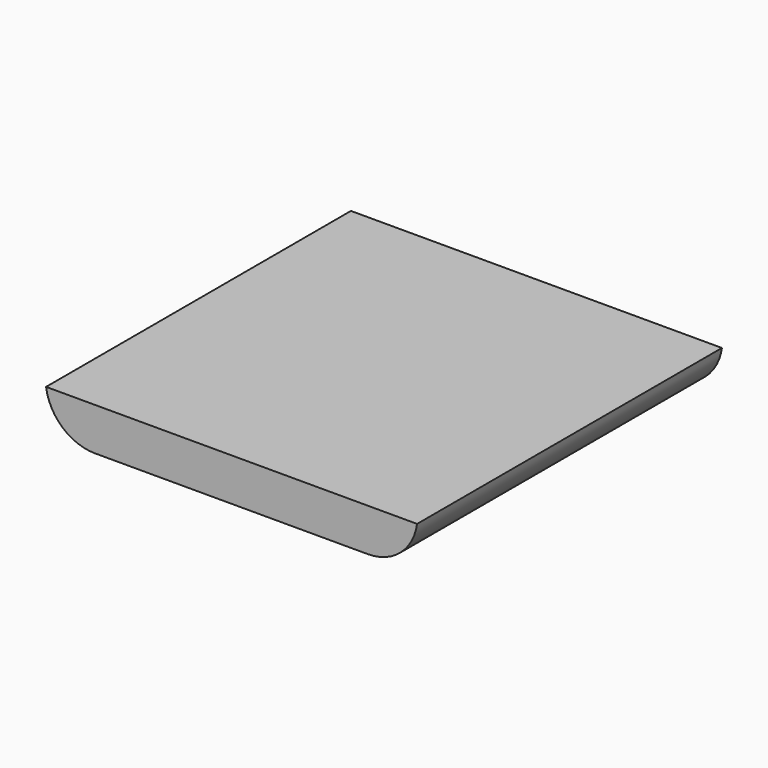
from build123d import *

# Parameters (mm, degrees)
F0_W        = 495.8
F0_H        = 509.2
F1_DEPTH    = 57
F2_T1_DEPTH = 836.1174207656


# Not quite as in the source:
# - a fillet or chamfer that OpenCascade refuses, or shapes differently, is made with other operations: its cross-section is extruded or revolved along the edge and cut away or added


with BuildPart() as f1:
    # F0 (on Top) → F1 (new body)
    with BuildSketch(Plane.XY):
        with Locations((247.9, -254.6)):
            Rectangle(F0_W, F0_H)
    extrude(amount=F1_DEPTH)

    # F2: fillet of radius 66 on 2 edges, made by hand

    # F2_s2 → F2_t1 (cut)
    with BuildSketch(Plane.XZ.offset(-163.4587103828)):
        with BuildLine():
            ThreePointArc((0, 57), (22.0129872687, 16.2506281447), (65.3834841531, 0))
            Line((65.3834841531, 0), (0, 0))
            Line((0, 0), (0, 57))
        make_face()
        with BuildLine():
            ThreePointArc((495.8, 57), (473.7870127313, 16.2506281447), (430.4165158469, 0))
            Line((430.4165158469, 0), (495.8, 0))
            Line((495.8, 0), (495.8, 57))
        make_face()
    extrude(amount=F2_T1_DEPTH, mode=Mode.SUBTRACT)


solid = f1.part
